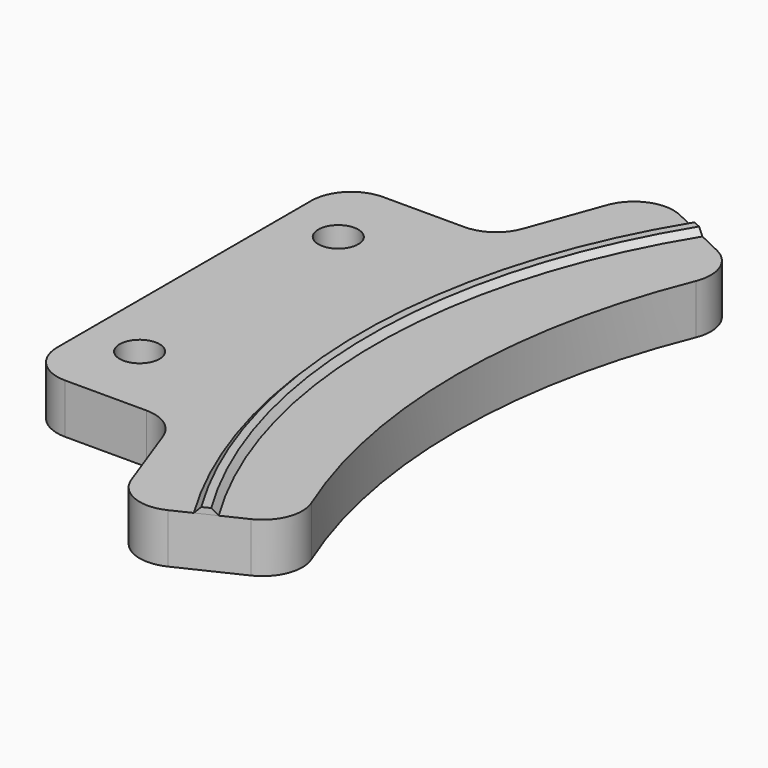
from build123d import *

# Parameters (mm, degrees)
F1_DEPTH = 6.35
F3_DEPTH = 0.762
F4_SIZE  = 0.76199
F5_R     = 2.5527
F6_DEPTH = 6.351
F7_R     = 5.08


# Not quite as in the source:
# - a fillet or chamfer is up to 0.001 mm smaller than in the source, because OpenCascade refuses the exact size


with BuildPart() as f1:
    # F0 (on Top) → F1 (new body)
    with BuildSketch(Plane.XY):
        with BuildLine():
            Line((19.05, 25.4), (0, 25.4))
            Line((0, 25.4), (0, -25.4))
            Line((0, -25.4), (19.05, -25.4))
            Line((19.05, -25.4), (25.5654837304, -43.301144426))
            Line((25.5654837304, -43.301144426), (42.7578812746, -35.0960261037))
            ThreePointArc((42.7578812746, -35.0960261037), (34.8122963703, 0), (42.7578812746, 35.0960261037))
            Line((42.7578812746, 35.0960261037), (25.5654837304, 43.301144426))
            Line((25.5654837304, 43.301144426), (19.05, 25.4))
        make_face()
    extrude(amount=F1_DEPTH)

    # F2 (on face) → F3 (join)
    with BuildSketch(Plane.XY.offset(6.35)):
        with BuildLine():
            Line((35.3141257953, 38.64857858), (33.0094497647, 39.7484914617))
            ThreePointArc((33.0094497647, 39.7484914617), (21.8558198534, 0), (33.0094497647, -39.7484914617))
            Line((33.0094497647, -39.7484914617), (35.3141257953, -38.64857858))
            ThreePointArc((35.3141257953, -38.64857858), (24.3958198534, 0), (35.3141257953, 38.64857858))
        make_face()
    extrude(amount=F3_DEPTH)

    # F4 (size 0.762 in the source; OpenCascade refuses exactly that, so slightly less here)
    f4_edges = [f1.edges().sort_by_distance(p)[0] for p in [
        (21.85582, 0, 7.112),
        (24.39582, 0, 7.112),
    ]]
    chamfer(f4_edges, length=F4_SIZE)

    # F5 (on face) → F6 (cut, through all)
    with BuildSketch(Plane.XY.offset(6.35)):
        with Locations((6.985, 15.875)):
            Circle(F5_R)
        with Locations((6.985, -15.875)):
            Circle(F5_R)
    extrude(amount=-F6_DEPTH, mode=Mode.SUBTRACT)

    # F7
    f7_edges = [f1.edges().sort_by_distance(p)[0] for p in [
        (0, -25.4, 3.175),
        (19.05, -25.4, 3.175),
        (25.565484, -43.301144, 3.175),
        (42.757881, -35.096026, 3.175),
        (0, 25.4, 3.175),
        (19.05, 25.4, 3.175),
        (25.565484, 43.301144, 3.175),
        (42.757881, 35.096026, 3.175),
    ]]
    fillet(f7_edges, radius=F7_R)


solid = f1.part
